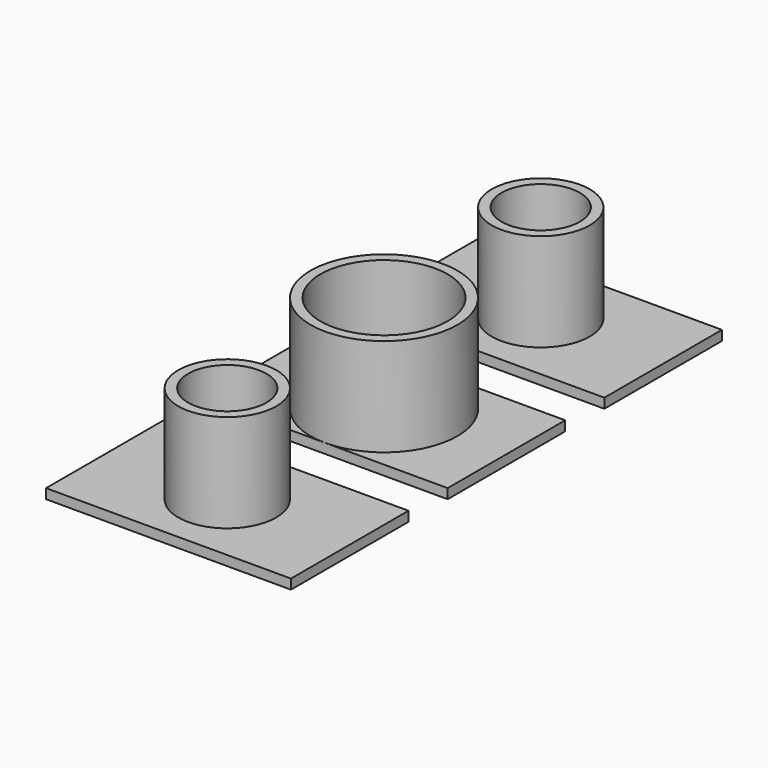
from build123d import *

# Parameters (mm, degrees)
F1_DEPTH = 2
F0_W     = 50
F0_H     = 30
F0_R     = 10
F0_R_2   = 13
F2_DEPTH = 22
F0_R_3   = 8


with BuildPart() as f1:
    # F0 (on Top) → F1 (new body)
    with BuildSketch(Plane.XY):
        with BuildLine():
            Line((0, 15), (-25, 15))
            Line((-25, 15), (-25, -15))
            Line((-25, -15), (3.27e-08, -15))
            ThreePointArc((3.27e-08, -15), (-15, -1.63e-08), (0, 15))
        make_face()
    extrude(amount=F1_DEPTH)



with BuildPart() as f1b:
    # F0 (on Top) → F1, piece 2 (new body)
    with BuildSketch(Plane.XY):
        with BuildLine():
            Line((25, 15), (0, 15))
            ThreePointArc((0, 15), (10.6066017178, 10.6066017178), (15, 0))
            ThreePointArc((15, 0), (10.6066017294, -10.6066017062), (3.27e-08, -15))
            Line((3.27e-08, -15), (25, -15))
            Line((25, -15), (25, 15))
        make_face()
    extrude(amount=F1_DEPTH)


with BuildPart() as f1c:
    # F0 (on Top) → F1, piece 3 (new body)
    with BuildSketch(Plane.XY):
        with Locations((0, 40)):
            Rectangle(F0_W, F0_H)
        with Locations((0, 40)):
            Circle(F0_R, mode=Mode.SUBTRACT)
    extrude(amount=F1_DEPTH)


with BuildPart() as f1d:
    # F0 (on Top) → F1, piece 4 (new body)
    with BuildSketch(Plane.XY):
        with Locations((0, -40)):
            Rectangle(F0_W, F0_H)
        with Locations((0, -40)):
            Circle(F0_R, mode=Mode.SUBTRACT)
    extrude(amount=F1_DEPTH)


with BuildPart() as f1_1:
    add(f1.part)

    add(f1b.part)  # F2 merges F1b
    # F0 (on Top) → F2 (join)
    with BuildSketch(Plane.XY):
        with BuildLine():
            ThreePointArc((15, 0), (10.6066017178, 10.6066017178), (0, 15))
            ThreePointArc((0, 15), (-15, -1.63e-08), (3.27e-08, -15))
            ThreePointArc((3.27e-08, -15), (10.6066017294, -10.6066017062), (15, 0))
        make_face()
        Circle(F0_R_2, mode=Mode.SUBTRACT)
    extrude(amount=F2_DEPTH)


with BuildPart() as f2:
    # F0 (on Top) → F2, piece 2 (new body)
    with BuildSketch(Plane.XY):
        with Locations((0, 40)):
            Circle(F0_R)
        with Locations((0, 40)):
            Circle(F0_R_3, mode=Mode.SUBTRACT)
    extrude(amount=F2_DEPTH)


with BuildPart() as f2b:
    # F0 (on Top) → F2, piece 3 (new body)
    with BuildSketch(Plane.XY):
        with Locations((0, -40)):
            Circle(F0_R)
        with Locations((0, -40)):
            Circle(F0_R_3, mode=Mode.SUBTRACT)
    extrude(amount=F2_DEPTH)


solid = Compound([f1c.part, f1d.part, f1_1.part, f2.part, f2b.part])
